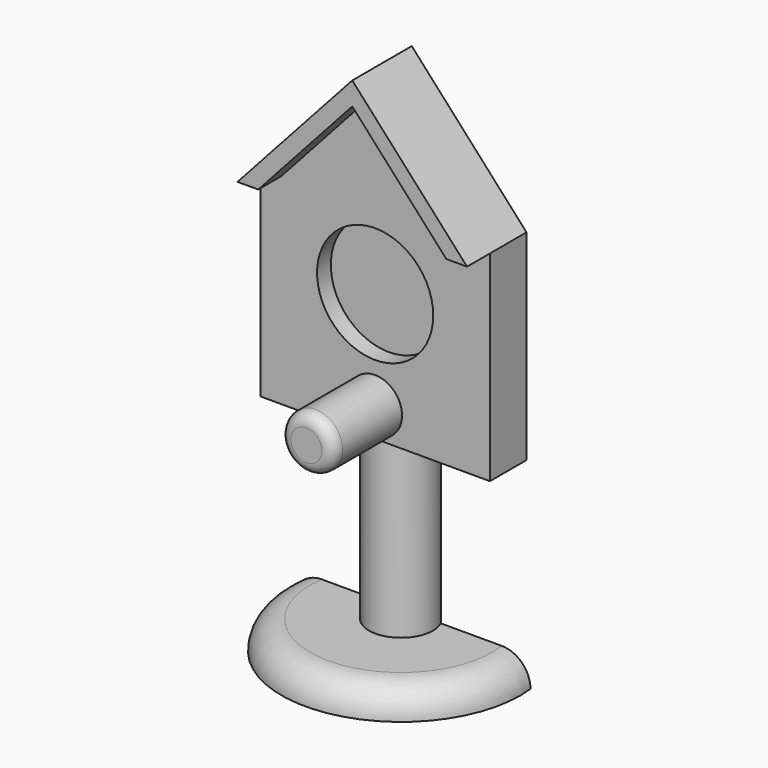
from build123d import *

# Parameters (mm, degrees)
F0_W      = 20.0620945543
F0_H      = 35.0510179996
F1_DEPTH  = 8
F2_R      = 10.1507039691
F3_DEPTH  = 3
F4_R      = 4.6971638308
F5_DEPTH  = 15
F6_R      = 2
F8_DEPTH  = 35
F10_DEPTH = 5
F11_R     = 4.99999
F13_DEPTH = 5


# Not quite as in the source:
# - a fillet or chamfer is up to 0.001 mm smaller than in the source, because OpenCascade refuses the exact size


with BuildPart() as f1:
    # F0 (on Front) → F1 (new body)
    with BuildSketch(Plane.XZ):
        Polygon((0, 57.1884997189), (0, 35.0510179996), (20.0620945543, 35.0510179996), align=None)
        Polygon((-20.0620945543, 35.0510179996), (0, 35.0510179996), (0, 57.1884997189), align=None)
        with Locations((-10.0310472772, 17.5255089998)):
            Rectangle(F0_W, F0_H)
        with Locations((10.0310472772, 17.5255089998)):
            Rectangle(F0_W, F0_H)
    extrude(amount=F1_DEPTH)

    # F2 (on face) → F3 (cut)
    with BuildSketch(Plane.XZ.offset(8)):
        with Locations((0, 22.2692545503)):
            Circle(F2_R)
    extrude(amount=-F3_DEPTH, mode=Mode.SUBTRACT)

    # F4 (on face) → F5 (join)
    with BuildSketch(Plane.XZ.offset(8)):
        with Locations((0, 5.1159886643)):
            Circle(F4_R)
    extrude(amount=F5_DEPTH)

    # F6
    f6_edges = [f1.edges().sort_by_distance(p)[0] for p in [
        (-4.697164, -23, 5.115989),
    ]]
    fillet(f6_edges, radius=F6_R)

    # F7 (on face) → F8 (join)
    with BuildSketch(Plane(origin=(0, 0, 0), x_dir=(1, 0, 0), z_dir=(0, 0, -1))):
        with BuildLine():
            Line((-5.0843584387, 0), (5.0843584387, 0))
            ThreePointArc((5.0843584387, 0), (0, 7.9473265145), (-5.0843584387, 0))
        make_face()
    extrude(amount=F8_DEPTH)

    # F12 (on face) → F13 (join)
    with BuildSketch(Plane.XZ.offset(8)):
        Polygon((0, 57.1884997189), (-20.0620945543, 35.0510179996), (-16.4370942388, 35.0510179996), (0, 53.1884997189), (16.4370942388, 35.0510179996), (20.0620945543, 35.0510179996), align=None)
    extrude(amount=F13_DEPTH)


with BuildPart() as f10:
    # F9 (on face) → F10 (new body)
    with BuildSketch(Plane(origin=(0, 0, -35), x_dir=(1, 0, 0), z_dir=(0, 0, -1))):
        with BuildLine():
            Line((5.0843584387, 0), (20.7567422331, 0))
            ThreePointArc((20.7567422331, 0), (0, 23.2363286774), (-20.7567422331, 0))
            Line((-20.7567422331, 0), (-5.0843584387, 0))
            ThreePointArc((-5.0843584387, 0), (0, 7.9473265145), (5.0843584387, 0))
        make_face()
    extrude(amount=-F10_DEPTH)

    # F11 (radius 5 in the source; OpenCascade refuses exactly that, so slightly less here)
    f11_edges = [f10.edges().sort_by_distance(p)[0] for p in [
        (0, -23.236329, -30),
    ]]
    fillet(f11_edges, radius=F11_R)


solid = Compound([f1.part, f10.part])
